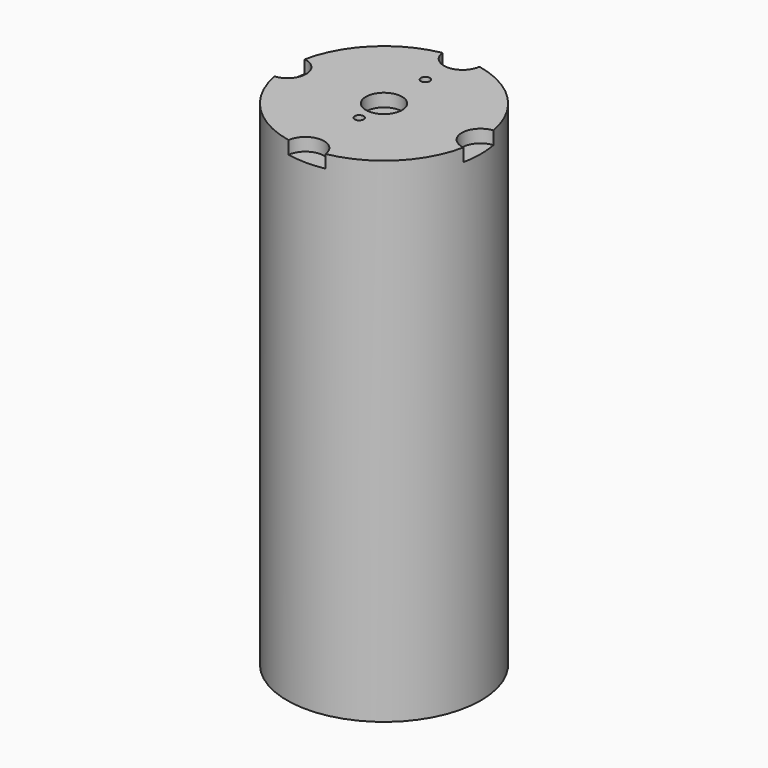
from build123d import *

# Parameters (mm, degrees)
F0_R     = 9.525
F0_R_2   = 0.4445
F1_DEPTH = 2.54
F2_R     = 1.778
F3_DEPTH = 1.27
F4_R     = 9.525
F4_R_2   = 5.4
F5_DEPTH = 46


# Not quite as in the source:
# - a feature names something its author has since deleted; it is built from what else it names


with BuildPart() as f1:
    # F0 (on Top) → F1 (new body)
    with BuildSketch(Plane.XY):
        Circle(F0_R)
        with Locations((0, -3.0520705041)):
            Circle(F0_R_2, mode=Mode.SUBTRACT)
        with Locations((0, 5.08)):
            Circle(F0_R_2, mode=Mode.SUBTRACT)
    extrude(amount=F1_DEPTH)

    # F2 (on face) → F3 (cut)
    with BuildSketch(Plane.XY.offset(2.54)):
        Circle(F2_R)
        with BuildLine():
            ThreePointArc((9.525, 0), (9.4846037847, 0.876308192), (9.3637577853, 1.7451834108))
            ThreePointArc((9.3637577853, 1.7451834108), (7.7122697392, -0.0678733407), (9.3315921315, -1.9097155001))
            ThreePointArc((9.3315921315, -1.9097155001), (9.4765246808, -0.9597421392), (9.525, 0))
        make_face()
        with BuildLine():
            ThreePointArc((-1.7451834108, 9.3637577853), (0.0678733407, 7.7122697392), (1.9097155001, 9.3315921315))
            ThreePointArc((1.9097155001, 9.3315921315), (0.0838233823, 9.5246311551), (-1.7451834108, 9.3637577853))
        make_face()
        with BuildLine():
            ThreePointArc((-1.9097155001, -9.3315921315), (-0.0838233823, -9.5246311551), (1.7451834108, -9.3637577853))
            ThreePointArc((1.7451834108, -9.3637577853), (-0.0678733407, -7.7122697392), (-1.9097155001, -9.3315921315))
        make_face()
        with BuildLine():
            ThreePointArc((-9.3637577853, -1.7451834108), (-7.7122697392, 0.0678733407), (-9.3315921315, 1.9097155001))
            ThreePointArc((-9.3315921315, 1.9097155001), (-9.5246311551, 0.0838233823), (-9.3637577853, -1.7451834108))
        make_face()
    extrude(amount=-F3_DEPTH, mode=Mode.SUBTRACT)

    # F4 (on face) → F5 (join)
    with BuildSketch(Plane(origin=(0, 0, 0), x_dir=(1, 0, 0), z_dir=(0, 0, -1))):
        Circle(F4_R)
        with BuildLine():
            ThreePointArc((5.0657137645, 6.9156561732), (7.6457042676, 3.8769785274), (8.5725, 0))
            ThreePointArc((8.5725, 0), (-3.8769785274, -7.6457042676), (-5.0657137645, 6.9156561732))
            ThreePointArc((-5.0657137645, 6.9156561732), (0, 9.4230005905), (5.0657137645, 6.9156561732))
        make_face(mode=Mode.SUBTRACT)
        with BuildLine():
            ThreePointArc((6.3709300865, 3.0520705041), (6.0358122236, 5.0911195392), (5.0657137645, 6.9156561732))
            ThreePointArc((5.0657137645, 6.9156561732), (0, 8.5725), (-5.0657137645, 6.9156561732))
            ThreePointArc((-5.0657137645, 6.9156561732), (-2.0390490351, -2.9837417196), (6.3709300865, 3.0520705041))
        make_face()
        with Locations((0, 3.0520705041)):
            Circle(F4_R_2, mode=Mode.SUBTRACT)
        with BuildLine():
            ThreePointArc((-5.0657137645, 6.9156561732), (0, 8.5725), (5.0657137645, 6.9156561732))
            ThreePointArc((5.0657137645, 6.9156561732), (0, 9.4230005905), (-5.0657137645, 6.9156561732))
        make_face()
    extrude(amount=F5_DEPTH)


solid = f1.part
